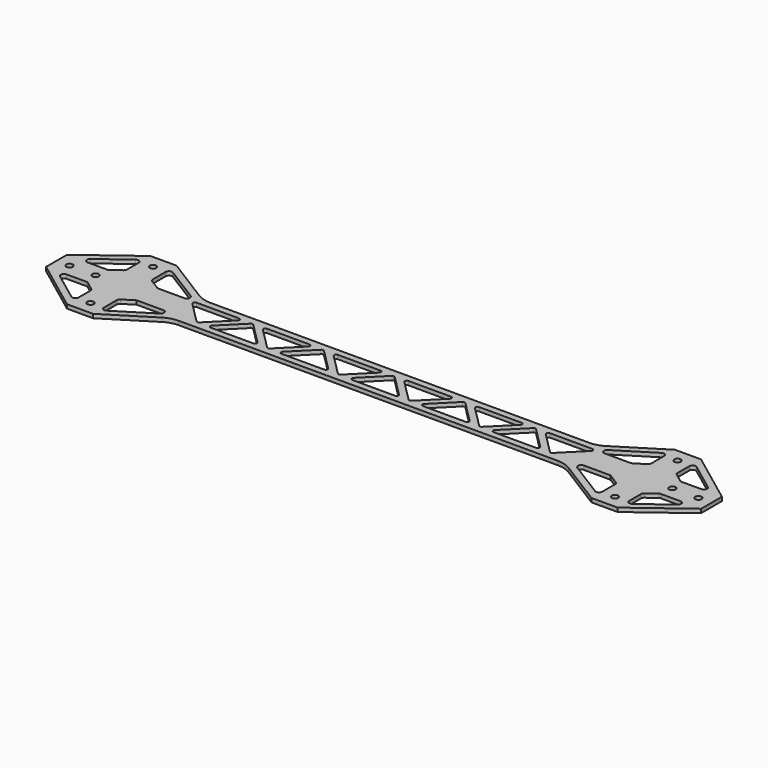
from build123d import *

# Parameters (mm, degrees)
F1_DEPTH = 3


# Not quite as in the source:
# - ends of sketch curves that miss each other by under 0.0002 mm in the source are joined


with BuildPart() as f1:
    # F0 (on Top) → F1 (new body)
    with BuildSketch(Plane.XY):
        with BuildLine():
            Line((-211, -40), (-191, -40))
            Line((-191, -40), (-155.863841, -18.039901))
            ThreePointArc((-155.863841, -18.039901), (-150.7424132157, -15.7648604604), (-145.1908530009, -15.0000002583))
            Line((-145.1908530009, -15.0000002583), (145.2644, -15))
            ThreePointArc((145.2644, -15), (150.7381727568, -15.7636330923), (155.7939501119, -17.9962188193))
            Line((155.7939501119, -17.9962188193), (191, -40))
            Line((191, -40), (211, -40))
            Line((211, -40), (251, -10))
            Line((251, -10), (251, 10))
            Line((251, 10), (211, 40))
            Line((211, 40), (191, 40))
            Line((191, 40), (155.863764, 18.039852))
            ThreePointArc((155.863764, 18.039852), (150.7364504809, 15.7631360477), (145.1785369986, 14.9999996814))
            Line((145.1785369986, 14.9999996814), (-145.2644, 15))
            ThreePointArc((-145.2644, 15), (-150.8179040565, 15.7864997282), (-155.9346251699, 18.0841407306))
            Line((-155.9346251699, 18.0841407306), (-191, 40))
            Line((-191, 40), (-211, 40))
            Line((-211, 40), (-251, 10))
            Line((-251, 10), (-251, -10))
            Line((-251, -10), (-211, -40))
        make_face()
        with BuildLine():
            ThreePointArc((-203.5, -30), (-202.767766953, -28.232233047), (-201, -27.5))
            ThreePointArc((-201, -27.5), (-199.232233047, -28.232233047), (-198.5, -30))
            ThreePointArc((-198.5, -30), (-199.232233047, -31.767766953), (-201, -32.5))
            ThreePointArc((-201, -32.5), (-202.767766953, -31.767766953), (-203.5, -30))
        make_face(mode=Mode.SUBTRACT)
        with BuildLine():
            ThreePointArc((-211, -28.753468), (-212.3855523171, -30.9913255384), (-215.0064050896, -30.7486481187))
            Line((-215.0064050896, -30.7486481187), (-236.688095, -14.500571))
            ThreePointArc((-236.688095, -14.500571), (-237.5594673422, -11.7060807046), (-235.1808639995, -9.9999998321))
            Line((-235.1808639995, -9.9999998321), (-220.132169, -10))
            ThreePointArc((-220.132169, -10), (-219.3435120087, -10.1276551368), (-218.6353959103, -10.4975838799))
            ThreePointArc((-218.6353959103, -10.4975838799), (-218.6311184846, -10.5007883178), (-218.6268479192, -10.5040018929))
            Line((-218.6268479192, -10.5040018929), (-211.998927, -15.480386))
            ThreePointArc((-211.998927, -15.480386), (-211.2612633974, -16.3668719989), (-211.0000002606, -17.4901469989))
            Line((-211.0000002606, -17.4901469989), (-211, -28.753468))
        make_face(mode=Mode.SUBTRACT)
        with BuildLine():
            Line((-189.815712, -15.155876), (-181.564585, -10))
            Line((-181.564585, -10), (-161.150958, -10))
            ThreePointArc((-161.150958, -10), (-158.7469997573, -11.8137167005), (-159.8311208842, -14.6232121862))
            Line((-159.8311208842, -14.6232121862), (-187.175019, -31.713149))
            ThreePointArc((-187.175019, -31.713149), (-189.7158714501, -31.7775740959), (-190.9999998, -29.5841530007))
            Line((-190.9999998, -29.5841530007), (-191, -17.281647))
            ThreePointArc((-191, -17.281647), (-190.6839505365, -16.0649465216), (-189.815712, -15.155876))
        make_face(mode=Mode.SUBTRACT)
        with BuildLine():
            ThreePointArc((-90.9669898368, -7.4394818368), (-90.6428905106, -9.0762597686), (-92.0324179995, -9.9999998451))
            Line((-92.0324179995, -9.9999998451), (-124.780739, -10))
            ThreePointArc((-124.780739, -10), (-126.1652980455, -9.0770582722), (-125.8460340007, -7.4439949993))
            Line((-125.8460340007, -7.4439949993), (-109.462826, 8.939213))
            ThreePointArc((-109.462826, 8.939213), (-108.3992389256, 9.3785491441), (-107.3373749037, 8.9350650956))
            Line((-107.3373749037, 8.9350650956), (-90.9669898368, -7.4394818368))
        make_face(mode=Mode.SUBTRACT)
        with BuildLine():
            ThreePointArc((-36.7956753368, -7.4351573367), (-36.4717506212, -9.0723564274), (-37.8620150028, -9.9956727509))
            Line((-37.8620150028, -9.9956727509), (-70.609427, -9.995672))
            ThreePointArc((-70.609427, -9.995672), (-71.9939859089, -9.0727305999), (-71.6747225007, -7.4396675037))
            Line((-71.6747225007, -7.4396675037), (-55.291519, 8.943535))
            ThreePointArc((-55.291519, 8.943535), (-54.2290346631, 9.3828738906), (-53.167621966, 8.9409520338))
            Line((-53.167621966, 8.9409520338), (-36.7956753368, -7.4351573367))
        make_face(mode=Mode.SUBTRACT)
        with BuildLine():
            ThreePointArc((17.4330091632, -7.4265068368), (17.7567238176, -9.0642083725), (16.3655799985, -9.9870173299))
            Line((16.3655799985, -9.9870173299), (-16.380747, -9.987017))
            ThreePointArc((-16.380747, -9.987017), (-17.7678199074, -9.0580062726), (-17.4367520007, -7.4217219993))
            Line((-17.4367520007, -7.4217219993), (-1.062835, 8.952195))
            ThreePointArc((-1.062835, 8.952195), (0.0006604442, 9.391532322), (1.0624875975, 8.948178593))
            Line((1.0624875975, 8.948178593), (17.4330091632, -7.4265068368))
        make_face(mode=Mode.SUBTRACT)
        with BuildLine():
            Line((161.150958, -10), (181.564585, -10))
            Line((181.564585, -10), (189.815712, -15.155876))
            ThreePointArc((189.815712, -15.155876), (190.6839505365, -16.0649465216), (191, -17.281647))
            Line((191, -17.281647), (191, -29.584153))
            ThreePointArc((191, -29.584153), (189.7158714501, -31.7775740959), (187.1750190095, -31.7131489847))
            Line((187.1750190095, -31.7131489847), (159.831121, -14.623212))
            ThreePointArc((159.831121, -14.623212), (158.7469997573, -11.8137167005), (161.150958, -10))
        make_face(mode=Mode.SUBTRACT)
        with BuildLine():
            ThreePointArc((198.5, -30), (199.232233047, -28.232233047), (201, -27.5))
            ThreePointArc((201, -27.5), (202.767766953, -28.232233047), (203.5, -30))
            ThreePointArc((203.5, -30), (202.767766953, -31.767766953), (201, -32.5))
            ThreePointArc((201, -32.5), (199.232233047, -31.767766953), (198.5, -30))
        make_face(mode=Mode.SUBTRACT)
        with BuildLine():
            Line((236.688095, -14.500571), (215.006405, -30.748648))
            ThreePointArc((215.006405, -30.748648), (212.3855523171, -30.9913255384), (211, -28.753468))
            Line((211, -28.753468), (211, -17.490147))
            ThreePointArc((211, -17.490147), (211.2612633974, -16.3668719989), (211.9989268471, -15.4803857964))
            Line((211.9989268471, -15.4803857964), (218.626848, -10.504002))
            ThreePointArc((218.626848, -10.504002), (218.6311184846, -10.5007883178), (218.6353959103, -10.4975838799))
            ThreePointArc((218.6353959103, -10.4975838799), (219.3435120087, -10.1276551368), (220.132169, -10))
            Line((220.132169, -10), (235.180864, -10))
            ThreePointArc((235.180864, -10), (237.5594673422, -11.7060807046), (236.688095, -14.500571))
        make_face(mode=Mode.SUBTRACT)
        with BuildLine():
            ThreePointArc((37.75497, -9.995897), (36.3704110911, -9.0729555999), (36.6896744993, -7.4398925037))
            Line((36.6896744993, -7.4398925037), (53.072881, 8.943314))
            ThreePointArc((53.072881, 8.943314), (54.1311378951, 9.382651075), (55.1907967264, 8.9467067247))
            Line((55.1907967264, 8.9467067247), (71.568725, -7.435385))
            ThreePointArc((71.568725, -7.435385), (71.8948904064, -9.0671724887), (70.5140990013, -9.9958973144))
            Line((70.5140990013, -9.9958973144), (37.75497, -9.995897))
        make_face(mode=Mode.SUBTRACT)
        with BuildLine():
            ThreePointArc((91.926282, -9.99157), (90.5417229545, -9.0686282722), (90.8609869993, -7.4355649993))
            Line((90.8609869993, -7.4355649993), (107.244193, 8.947641))
            ThreePointArc((107.244193, 8.947641), (108.3024495416, 9.3869790745), (109.3621087264, 8.9510347247))
            Line((109.3621087264, 8.9510347247), (125.740036, -7.431057))
            ThreePointArc((125.740036, -7.431057), (126.0662015961, -9.0628440282), (124.6854109972, -9.9915693103))
            Line((124.6854109972, -9.9915693103), (91.926282, -9.99157))
        make_face(mode=Mode.SUBTRACT)
        with BuildLine():
            ThreePointArc((-243.5, 0), (-242.767766953, 1.767766953), (-241, 2.5))
            ThreePointArc((-241, 2.5), (-239.232233047, 1.767766953), (-238.5, 0))
            ThreePointArc((-238.5, 0), (-239.232233047, -1.767766953), (-241, -2.5))
            ThreePointArc((-241, -2.5), (-242.767766953, -1.767766953), (-243.5, 0))
        make_face(mode=Mode.SUBTRACT)
        with BuildLine():
            ThreePointArc((-223.5, 0), (-222.767766953, 1.767766953), (-221, 2.5))
            ThreePointArc((-221, 2.5), (-219.232233047, 1.767766953), (-218.5, 0))
            ThreePointArc((-218.5, 0), (-219.232233047, -1.767766953), (-221, -2.5))
            ThreePointArc((-221, -2.5), (-222.767766953, -1.767766953), (-223.5, 0))
        make_face(mode=Mode.SUBTRACT)
        with BuildLine():
            Line((-151.823704, 9.984309), (-119.0648, 9.984309))
            ThreePointArc((-119.0648, 9.984309), (-117.6838280624, 9.0556855873), (-118.0099508368, 7.4237948368))
            Line((-118.0099508368, 7.4237948368), (-134.388348, -8.958766))
            ThreePointArc((-134.388348, -8.958766), (-135.4478675094, -9.3942415038), (-136.5057916718, -8.9549036718))
            Line((-136.5057916718, -8.9549036718), (-152.879709, 7.419013))
            ThreePointArc((-152.879709, 7.419013), (-153.2107770414, 9.0552979471), (-151.823704, 9.984309))
        make_face(mode=Mode.SUBTRACT)
        with BuildLine():
            Line((-97.724254, 9.987017), (-64.977242, 9.987017))
            ThreePointArc((-64.977242, 9.987017), (-63.5866538517, 9.06388784), (-63.9105008368, 7.4265038368))
            Line((-63.9105008368, 7.4265038368), (-80.288898, -8.956058))
            ThreePointArc((-80.288898, -8.956058), (-81.3484178616, -9.3915325032), (-82.4063416718, -8.9521946718))
            Line((-82.4063416718, -8.9521946718), (-98.789549, 7.431012))
            ThreePointArc((-98.789549, 7.431012), (-99.1088130455, 9.0640752722), (-97.724254, 9.987017))
        make_face(mode=Mode.SUBTRACT)
        with BuildLine():
            Line((-43.495574, 9.995672), (-10.748562, 9.995672))
            ThreePointArc((-10.748562, 9.995672), (-9.3579738517, 9.07254284), (-9.6818208368, 7.4351588368))
            Line((-9.6818208368, 7.4351588368), (-26.060217, -8.947403))
            ThreePointArc((-26.060217, -8.947403), (-27.1197371532, -9.3828775045), (-28.1776611718, -8.9435401718))
            Line((-28.1776611718, -8.9435401718), (-44.551579, 7.430377))
            ThreePointArc((-44.551579, 7.430377), (-44.8826469074, 9.0666612726), (-43.495574, 9.995672))
        make_face(mode=Mode.SUBTRACT)
        with BuildLine():
            Line((-211.998931, 15.502663), (-218.652535, 10.506996))
            ThreePointArc((-218.652535, 10.506996), (-219.3657375813, 10.1301362117), (-220.161819, 10))
            Line((-220.161819, 10), (-235.166667, 10))
            ThreePointArc((-235.166667, 10), (-237.5383752451, 11.709430585), (-236.666667, 14.5))
            Line((-236.666667, 14.5), (-214.992605, 30.755546))
            ThreePointArc((-214.992605, 30.755546), (-212.377839681, 30.9840210489), (-211, 28.750021))
            Line((-211, 28.750021), (-211, 17.511387))
            ThreePointArc((-211, 17.511387), (-211.2614985827, 16.3886849935), (-211.998931, 15.502663))
        make_face(mode=Mode.SUBTRACT)
        with BuildLine():
            ThreePointArc((-159.8344118419, 14.6252692552), (-158.7464410037, 11.8155926425), (-161.150934, 10))
            Line((-161.150934, 10), (-180.858194, 10))
            ThreePointArc((-180.858194, 10), (-181.5423765031, 10.0954430133), (-182.1743186545, 10.3744845581))
            Line((-182.1743186545, 10.3744845581), (-189.824799, 15.155035))
            ThreePointArc((-189.824799, 15.155035), (-190.6870562164, 16.0640441543), (-191.0000001281, 17.2772430001))
            Line((-191.0000001281, 17.2772430001), (-191, 29.593154))
            ThreePointArc((-191, 29.593154), (-189.7149159972, 31.7780977338), (-187.1808167042, 31.7167724761))
            Line((-187.1808167042, 31.7167724761), (-159.8344118419, 14.6252692552))
        make_face(mode=Mode.SUBTRACT)
        with BuildLine():
            ThreePointArc((-203.5, 30), (-202.767766953, 31.767766953), (-201, 32.5))
            ThreePointArc((-201, 32.5), (-199.232233047, 31.767766953), (-198.5, 30))
            ThreePointArc((-198.5, 30), (-199.232233047, 28.232233047), (-201, 27.5))
            ThreePointArc((-201, 27.5), (-202.767766953, 28.232233047), (-203.5, 30))
        make_face(mode=Mode.SUBTRACT)
        with BuildLine():
            Line((10.712005, 9.988411), (43.458914, 9.988411))
            ThreePointArc((43.458914, 9.988411), (44.8495861498, 9.0653298402), (44.5257591632, 7.4278978368))
            Line((44.5257591632, 7.4278978368), (28.148869, -8.953155))
            ThreePointArc((28.148869, -8.953155), (27.088903519, -9.3901360709), (26.0299128282, -8.9507971718))
            Line((26.0299128282, -8.9507971718), (9.64671, 7.432406))
            ThreePointArc((9.64671, 7.432406), (9.3274459545, 9.0654692722), (10.712005, 9.988411))
        make_face(mode=Mode.SUBTRACT)
        with BuildLine():
            Line((80.129366, -8.948091), (63.74616, 7.435115))
            ThreePointArc((63.74616, 7.435115), (63.4268959545, 9.0681782722), (64.811455, 9.99112))
            Line((64.811455, 9.99112), (97.558245, 9.99112))
            ThreePointArc((97.558245, 9.99112), (98.9490134002, 9.0680944381), (98.6252086632, 7.4306073367))
            Line((98.6252086632, 7.4306073367), (82.247282, -8.951485))
            ThreePointArc((82.247282, -8.951485), (81.1876225416, -9.3874290745), (80.129366, -8.948091))
        make_face(mode=Mode.SUBTRACT)
        with BuildLine():
            Line((134.358046, -8.939436), (117.97484, 7.44377))
            ThreePointArc((117.97484, 7.44377), (117.6555770899, 9.0768335971), (119.040136, 9.999775))
            Line((119.040136, 9.999775), (151.786926, 9.999775))
            ThreePointArc((151.786926, 9.999775), (153.1776944002, 9.0767494381), (152.8538896632, 7.4392623367))
            Line((152.8538896632, 7.4392623367), (136.475962, -8.942829))
            ThreePointArc((136.475962, -8.942829), (135.4163031858, -9.3787740739), (134.358046, -8.939436))
        make_face(mode=Mode.SUBTRACT)
        with BuildLine():
            ThreePointArc((218.5, 0), (219.232233047, 1.767766953), (221, 2.5))
            ThreePointArc((221, 2.5), (222.767766953, 1.767766953), (223.5, 0))
            ThreePointArc((223.5, 0), (222.767766953, -1.767766953), (221, -2.5))
            ThreePointArc((221, -2.5), (219.232233047, -1.767766953), (218.5, 0))
        make_face(mode=Mode.SUBTRACT)
        with BuildLine():
            ThreePointArc((238.5, 0), (239.232233047, 1.767766953), (241, 2.5))
            ThreePointArc((241, 2.5), (242.767766953, 1.767766953), (243.5, 0))
            ThreePointArc((243.5, 0), (242.767766953, -1.767766953), (241, -2.5))
            ThreePointArc((241, -2.5), (239.232233047, -1.767766953), (238.5, 0))
        make_face(mode=Mode.SUBTRACT)
        with BuildLine():
            Line((180.858194, 10), (161.150934, 10))
            ThreePointArc((161.150934, 10), (158.7464410037, 11.8155926425), (159.8344118419, 14.6252692552))
            Line((159.8344118419, 14.6252692552), (187.180817, 31.716772))
            ThreePointArc((187.180817, 31.716772), (189.7149159972, 31.7780977338), (191, 29.593154))
            Line((191, 29.593154), (191, 17.277243))
            ThreePointArc((191, 17.277243), (190.6870562164, 16.0640441543), (189.8247991531, 15.1550347549))
            Line((189.8247991531, 15.1550347549), (182.174319, 10.374484))
            ThreePointArc((182.174319, 10.374484), (181.5423765031, 10.0954430133), (180.858194, 10))
        make_face(mode=Mode.SUBTRACT)
        with BuildLine():
            ThreePointArc((220.161819, 10), (219.3657375813, 10.1301362117), (218.6525353787, 10.5069965001))
            Line((218.6525353787, 10.5069965001), (211.998931, 15.502663))
            ThreePointArc((211.998931, 15.502663), (211.2614985827, 16.3886849935), (211.0000000957, 17.5113869996))
            Line((211.0000000957, 17.5113869996), (211, 28.750021))
            ThreePointArc((211, 28.750021), (212.377839681, 30.9840210489), (214.9926049747, 30.755545966))
            Line((214.9926049747, 30.755545966), (236.666667, 14.5))
            ThreePointArc((236.666667, 14.5), (237.5383752451, 11.709430585), (235.166667, 10))
            Line((235.166667, 10), (220.161819, 10))
        make_face(mode=Mode.SUBTRACT)
        with BuildLine():
            ThreePointArc((198.5, 30), (199.232233047, 31.767766953), (201, 32.5))
            ThreePointArc((201, 32.5), (202.767766953, 31.767766953), (203.5, 30))
            ThreePointArc((203.5, 30), (202.767766953, 28.232233047), (201, 27.5))
            ThreePointArc((201, 27.5), (199.232233047, 28.232233047), (198.5, 30))
        make_face(mode=Mode.SUBTRACT)
    extrude(amount=F1_DEPTH)


solid = f1.part
